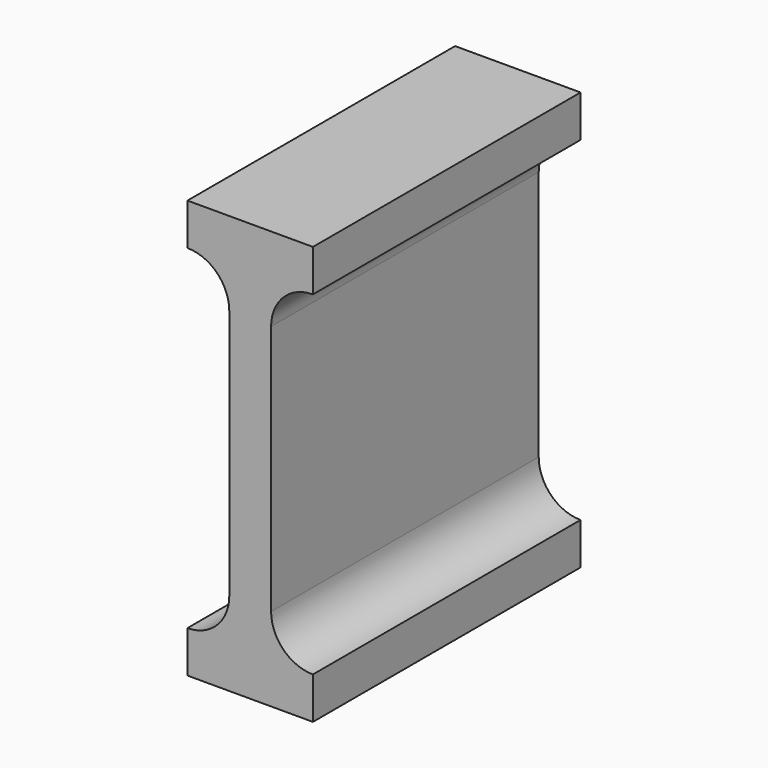
from build123d import *

# Parameters (mm, degrees)
F1_DEPTH = 40
F2_R     = 4.99999


# Not quite as in the source:
# - a fillet or chamfer is up to 0.001 mm smaller than in the source, because OpenCascade refuses the exact size


with BuildPart() as f1:
    # F0 (on Front) → F1 (new body)
    with BuildSketch(Plane.XZ):
        Polygon((-10.2562157065, 50), (-25.2562157065, 50), (-25.2562157065, 45), (-20.2562157065, 45), (-20.2562157065, 5), (-25.2562157065, 5), (-25.2562157065, 0), (-10.2562157065, 0), (-10.2562157065, 5), (-15.2562157065, 5), (-15.2562157065, 45), (-10.2562157065, 45), align=None)
    extrude(amount=F1_DEPTH)

    # F2 (radius 5 in the source; OpenCascade refuses exactly that, so slightly less here)
    f2_edges = [f1.edges().sort_by_distance(p)[0] for p in [
        (-15.256216, -20, 5),
        (-20.256216, -20, 5),
        (-15.256216, -20, 45),
        (-20.256216, -20, 45),
    ]]
    fillet(f2_edges, radius=F2_R)


solid = f1.part
